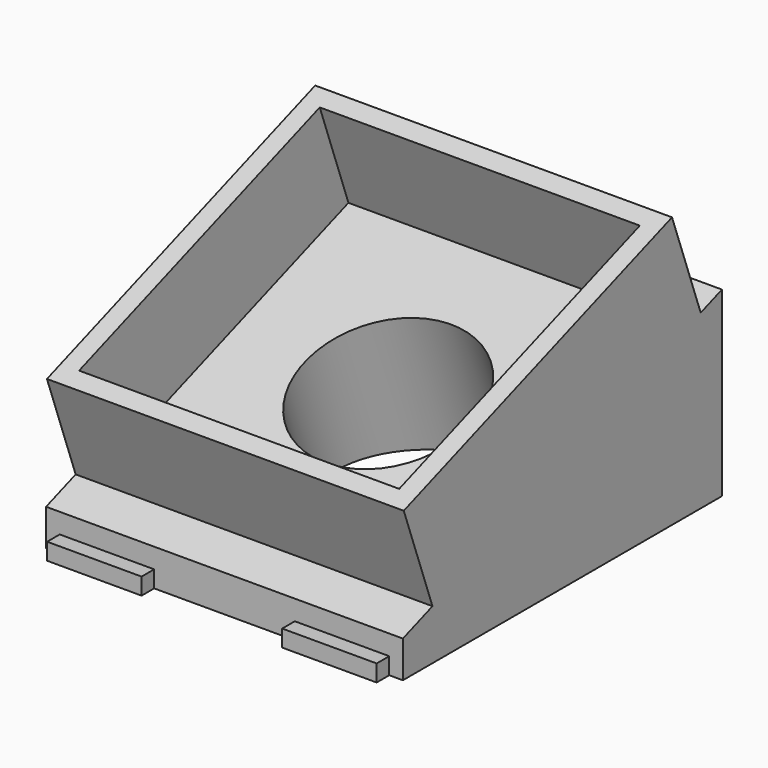
from build123d import *

# Parameters (mm, degrees)
F1_DEPTH = 1.6
F3_DEPTH = 20
F5_DEPTH = 34.001
F6_W     = 34
F6_H     = 34
F6_W_2   = 30.5
F6_H_2   = 30.5
F7_DEPTH = 10
F6_R     = 8
F8_DEPTH = 16.7997198341


# Not quite as in the source:
# - a feature names something its author has since deleted; it is built from what else it names


with BuildPart() as f1:
    # F0 (on Top) → F1 (new body)
    with BuildSketch(Plane.XY):
        Polygon((-15.7, 19), (-17, 19), (-17, -19), (-15.7, -19), (-15.7, -20.5), (-6.7, -20.5), (-6.7, -19), (6.7, -19), (6.7, -20.5), (15.7, -20.5), (15.7, -19), (17, -19), (17, 19), (15.7, 19), (15.7, 20.5), (6.7, 20.5), (6.7, 19), (-6.7, 19), (-6.7, 20.5), (-15.7, 20.5), align=None)
    extrude(amount=F1_DEPTH)

    # F2 (on face) → F3 (join)
    with BuildSketch(Plane.XY.offset(1.6)):
        Polygon((-15.7, 19), (-17, 19), (-17, -19), (-15.7, -19), (-6.7, -19), (6.7, -19), (15.7, -19), (17, -19), (17, 19), (15.7, 19), (6.7, 19), (-6.7, 19), align=None)
    extrude(amount=F3_DEPTH)

    # F4 (on face) → F5 (cut, through all)
    with BuildSketch(Plane(origin=(-17, 0, 0), x_dir=(0, -1, 0), z_dir=(-1, 0, 0))):
        Polygon((-19, 17.3308689021), (19, 3.5), (19, 21.6), (-19, 21.6), align=None)
    extrude(amount=-F5_DEPTH, mode=Mode.SUBTRACT)

    # F6 (on face) → F7 (join)
    with BuildSketch(Plane(origin=(0, -3.3474561073, 9.1970600675), x_dir=(1, 0, 0), z_dir=(0, -0.3420201433, 0.9396926208))):
        with Locations((0, 4.0929107067)):
            Rectangle(F6_W, F6_H)
        with Locations((0, 4.0929107067)):
            Rectangle(F6_W_2, F6_H_2, mode=Mode.SUBTRACT)
    extrude(amount=F7_DEPTH)

    # F6 (on face) → F8 (cut, through all)
    with BuildSketch(Plane(origin=(0, -3.3474561073, 9.1970600675), x_dir=(1, 0, 0), z_dir=(0, -0.3420201433, 0.9396926208))):
        with Locations((0, 4.0929107067)):
            Circle(F6_R)
    extrude(amount=-F8_DEPTH, mode=Mode.SUBTRACT)


solid = f1.part
